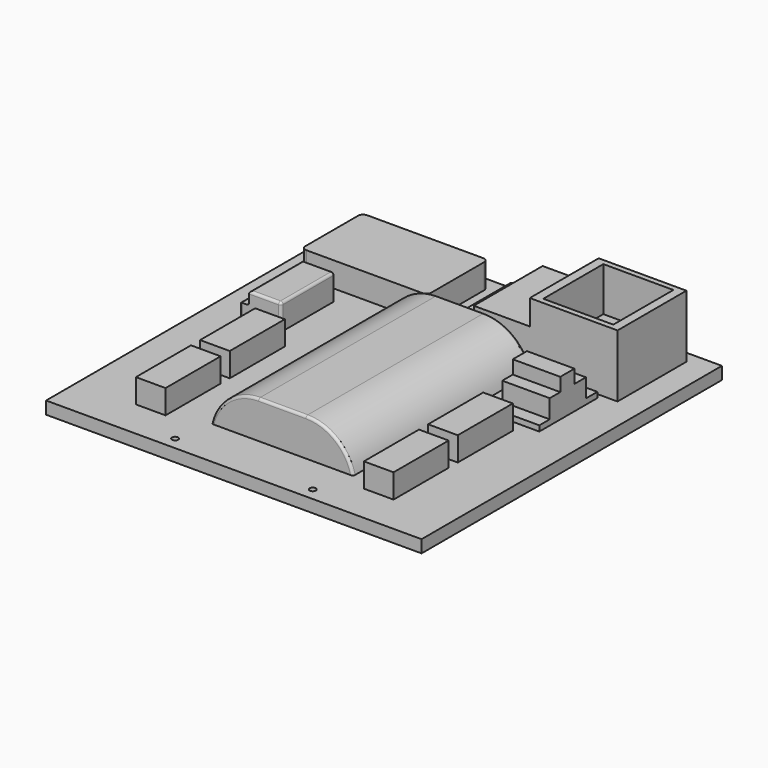
from build123d import *

# Parameters (mm, degrees)
F0_W         = 381
F0_H         = 381
F1_DEPTH     = 12.7
F3_W         = 144.018
F3_H         = 226.568
F4_DEPTH     = 38.1
F5_W         = 178.054
F5_H         = 87.376
F6_DEPTH     = 63.5
F7_W         = 127.762
F7_H         = 76.962
F8_DEPTH     = 25.146
F9_W         = 41.91
F9_H         = 68.1736
F10_DEPTH    = 26.035
F11_W        = 48.1622978261
F11_H        = 73.66
F12_DEPTH    = 38.1
F13_W        = 30.099
F13_H        = 69.85
F14_DEPTH    = 24.384
F15_T4_DEPTH = 466.4836595949
F15_T9_DEPTH = 466.4836595949
F16_W        = 71.074873209
F16_H        = 76.1698335409
F17_DEPTH    = 44.69176
F18_W        = 89.027
F18_H        = 87.376
F19_DEPTH    = 25.4
F20_W        = 32.1671016191
F20_H        = 87.376
F21_DEPTH    = 25.4
F22_W        = 48.1622978261
F22_H        = 29.0787754375
F22_H_2      = 26.581694724
F23_DEPTH    = 13.65146
F24_W        = 48.1622978261
F24_H        = 14.5393877187
F24_H_2      = 14.3073135987
F25_DEPTH    = 18.87303
F26_W        = 9.4362943637
F26_H        = 68.1736
F27_DEPTH    = 12.7
F28_R        = 2.54
F30_D        = 6.35
F31_R        = 5.08


# Not quite as in the source:
# - a fillet or chamfer that OpenCascade refuses, or shapes differently, is made with other operations: its cross-section is extruded or revolved along the edge and cut away or added


with BuildPart() as f1:
    # F0 (on Top) → F1 (new body)
    with BuildSketch(Plane.XY):
        Rectangle(F0_W, F0_H)
    extrude(amount=F1_DEPTH)

    # F3 (on face) → F4 (join)
    with BuildSketch(Plane.XY.offset(12.7)):
        with Locations((8.509, -26.416)):
            Rectangle(F3_W, F3_H)
    extrude(amount=F4_DEPTH)

    # F5 (on face) → F6 (join)
    with BuildSketch(Plane.XY.offset(12.7)):
        with Locations((75.1363011077, 134.6866802573)):
            Rectangle(F5_W, F5_H)
    extrude(amount=F6_DEPTH)

    # F7 (on face) → F8 (join)
    with BuildSketch(Plane.XY.offset(12.7)):
        with Locations((-101.4716736972, 140.4740017718)):
            Rectangle(F7_W, F7_H)
    extrude(amount=F8_DEPTH)

    # F9 (on face) → F10 (join)
    with BuildSketch(Plane.XY.offset(12.7)):
        with Locations((-139.3904201686, 51.5634464747)):
            Rectangle(F9_W, F9_H)
    extrude(amount=F10_DEPTH)

    # F11 (on face) → F12 (join)
    with BuildSketch(Plane.XY.offset(12.7)):
        with Locations((123.9150092006, 48.8317962736)):
            Rectangle(F11_W, F11_H)
    extrude(amount=F12_DEPTH)

    # F13 (on face) → F14 (join)
    with BuildSketch(Plane.XY.offset(12.7)):
        with Locations((-115.685201868, -34.925)):
            Rectangle(F13_W, F13_H)
        with Locations((-115.685201868, -116.3742716573)):
            Rectangle(F13_W, F13_H)
        with Locations((115.685201868, -34.925)):
            Rectangle(F13_W, F13_H)
        with Locations((115.685201868, -116.3742716573)):
            Rectangle(F13_W, F13_H)
    extrude(amount=F14_DEPTH)

    # F15: fillet of radius 49.2649730808 on 2 edges, made by hand


with BuildPart() as f15_tool2:
    # F15_s3 → F15_t4 (new body)
    with BuildSketch(Plane.XZ.offset(259.6578297975)):
        with BuildLine():
            ThreePointArc((80.518, 12.7), (63.1697785132, 40.1166266199), (32.534868081, 50.8))
            Line((32.534868081, 50.8), (80.518, 50.8))
            Line((80.518, 50.8), (80.518, 12.7))
        make_face()
    extrude(amount=-F15_T4_DEPTH)

    split(bisect_by=Plane.XZ.offset(-90.9986802573), keep=Keep.TOP)


with BuildPart() as f1_1:
    add(f1.part)

    # F15_t1: cut F15_tool2
    add(f15_tool2.part, mode=Mode.SUBTRACT)


with BuildPart() as f15_tool7:
    # F15_s8 → F15_t9 (new body)
    with BuildSketch(Plane.XZ.offset(-206.8258297975)):
        with BuildLine():
            ThreePointArc((-63.5, 12.7), (-46.1517785132, 40.1166266199), (-15.516868081, 50.8))
            Line((-15.516868081, 50.8), (-63.5, 50.8))
            Line((-63.5, 50.8), (-63.5, 12.7))
        make_face()
    extrude(amount=F15_T9_DEPTH)

    split(bisect_by=Plane.XZ.offset(-101.9930017718), keep=Keep.TOP)


with BuildPart() as f1_2:
    add(f1_1.part)

    # F15_t6: cut F15_tool7
    add(f15_tool7.part, mode=Mode.SUBTRACT)

    # F16 (on face) → F17 (cut)
    with BuildSketch(Plane.XY.offset(76.2)):
        with Locations((119.8119372129, 134.7657069564)):
            Rectangle(F16_W, F16_H)
    extrude(amount=-F17_DEPTH, mode=Mode.SUBTRACT)

    # F18 (on face) → F19 (cut)
    with BuildSketch(Plane.XY.offset(76.2)):
        with Locations((30.6228011077, 134.6866802573)):
            Rectangle(F18_W, F18_H)
    extrude(amount=-F19_DEPTH, mode=Mode.SUBTRACT)

    # F20 (on face) → F21 (cut)
    with BuildSketch(Plane.XY.offset(50.8)):
        with Locations((2.1928519172, 134.6866802573)):
            Rectangle(F20_W, F20_H)
    extrude(amount=-F21_DEPTH, mode=Mode.SUBTRACT)

    # F22 (on face) → F23 (cut)
    with BuildSketch(Plane.XY.offset(50.8)):
        with Locations((123.9150092006, 71.1224085549)):
            Rectangle(F22_W, F22_H)
        with Locations((123.9150092006, 25.2926436356)):
            Rectangle(F22_W, F22_H_2)
    extrude(amount=-F23_DEPTH, mode=Mode.SUBTRACT)

    # F24 (on face) → F25 (cut)
    with BuildSketch(Plane.XY.offset(37.14854)):
        with Locations((123.9150092006, 78.3921024142)):
            Rectangle(F24_W, F24_H)
        with Locations((123.9150092006, 18.045573961)):
            Rectangle(F24_W, F24_H_2)
    extrude(amount=-F25_DEPTH, mode=Mode.SUBTRACT)

    # F26 (on face) → F27 (cut)
    with BuildSketch(Plane.XY.offset(38.735)):
        with Locations((-155.6272729868, 51.5634464747)):
            Rectangle(F26_W, F26_H)
    extrude(amount=-F27_DEPTH, mode=Mode.SUBTRACT)

    # F28
    f28_edges = [f1_2.edges().sort_by_distance(p)[0] for p in [
        (-150.909126, 51.563446, 26.035),
        (-160.34542, 51.563446, 26.035),
        (-150.909126, 51.563446, 38.735),
        (-134.672273, 17.476646, 38.735),
        (-118.43542, 51.563446, 38.735),
        (-134.672273, 85.650246, 38.735),
        (-118.43542, 17.476646, 25.7175),
        (32.534868, -26.416, 50.8),
        (8.509, -139.7, 50.8),
        (-15.516868, -26.416, 50.8),
        (8.509, 86.868, 50.8),
        (-160.34542, 17.476646, 19.3675),
        (-160.34542, 85.650246, 19.3675),
        (-118.43542, 85.650246, 25.7175),
        (63.169779, 86.868, 40.116627),
        (63.169779, -139.7, 40.116627),
        (-46.151779, -139.7, 40.116627),
        (-46.151779, 86.868, 40.116627),
    ]]
    fillet(f28_edges, radius=F28_R)

    # F30 (through all)
    with Locations(Plane.XY.offset(12.7)):
        with Locations((-69.85, -177.6871830225), (69.85, -177.6871830225), (69.85, 184.4432204962), (-69.85, 184.4432204962)):
            Hole(F30_D / 2)

    # F31
    f31_edges = [f1_2.edges().sort_by_distance(p)[0] for p in [
        (-37.590674, 101.993002, 25.273),
        (-165.352674, 101.993002, 25.273),
        (-165.352674, 178.955002, 25.273),
        (-37.590674, 178.955002, 25.273),
    ]]
    fillet(f31_edges, radius=F31_R)


solid = f1_2.part
